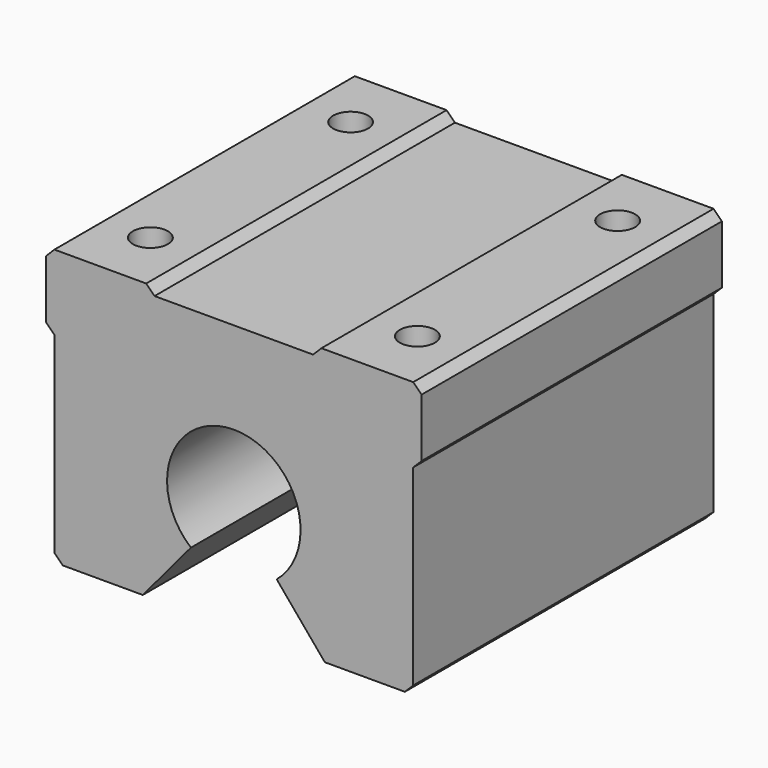
from build123d import *

# Parameters (mm, degrees)
F1_DEPTH = 45
F2_R     = 2.1
F3_DEPTH = 12
F4_SIZE  = 0.99999


# Not quite as in the source:
# - a fillet or chamfer is up to 0.001 mm smaller than in the source, because OpenCascade refuses the exact size


with BuildPart() as f1:
    # F0 (on Front) → F1 (new body)
    with BuildSketch(Plane.XZ):
        with BuildLine():
            Line((88.0538091608, -30.5978502929), (75.0538091608, -30.5978502929))
            Line((75.0538091608, -30.5978502929), (75.0538091608, -39.5978502929))
            Line((75.0538091608, -39.5978502929), (76.0538091608, -39.5978502929))
            Line((76.0538091608, -39.5978502929), (76.0538091608, -63.5978502929))
            Line((76.0538091608, -63.5978502929), (86.6455139554, -63.5978502929))
            Line((86.6455139554, -63.5978502929), (92.4115082833, -56.7262058379))
            ThreePointArc((92.4115082833, -56.7262058379), (97.5538091608, -42.5978502929), (102.6961100382, -56.7262058379))
            Line((102.6961100382, -56.7262058379), (108.4621043661, -63.5978502929))
            Line((108.4621043661, -63.5978502929), (119.0538091608, -63.5978502929))
            Line((119.0538091608, -63.5978502929), (119.0538091608, -39.5978502929))
            Line((119.0538091608, -39.5978502929), (120.0538091608, -39.5978502929))
            Line((120.0538091608, -39.5978502929), (120.0538091608, -30.5978502929))
            Line((120.0538091608, -30.5978502929), (107.0538091608, -30.5978502929))
            Line((107.0538091608, -30.5978502929), (107.0538091608, -31.5978502929))
            Line((107.0538091608, -31.5978502929), (88.0538091608, -31.5978502929))
            Line((88.0538091608, -31.5978502929), (88.0538091608, -30.5978502929))
        make_face()
    extrude(amount=F1_DEPTH)

    # F2 (on face) → F3 (cut)
    with BuildSketch(Plane.XY.offset(-30.5978502929)):
        with Locations((81.5538091608, -7.5)):
            Circle(F2_R)
        with Locations((81.5538091608, -37.5)):
            Circle(F2_R)
        with Locations((113.5538091608, -7.5)):
            Circle(F2_R)
        with Locations((113.5538091608, -37.5)):
            Circle(F2_R)
    extrude(amount=-F3_DEPTH, mode=Mode.SUBTRACT)

    # F4 (size 1 in the source; OpenCascade refuses exactly that, so slightly less here)
    f4_edges = [f1.edges().sort_by_distance(p)[0] for p in [
        (88.053809, -22.5, -30.59785),
        (107.053809, -22.5, -30.59785),
        (75.053809, -22.5, -30.59785),
        (75.053809, -22.5, -39.59785),
        (120.053809, -22.5, -30.59785),
        (120.053809, -22.5, -39.59785),
        (76.053809, -22.5, -63.59785),
        (119.053809, -22.5, -63.59785),
    ]]
    chamfer(f4_edges, length=F4_SIZE)


solid = f1.part
